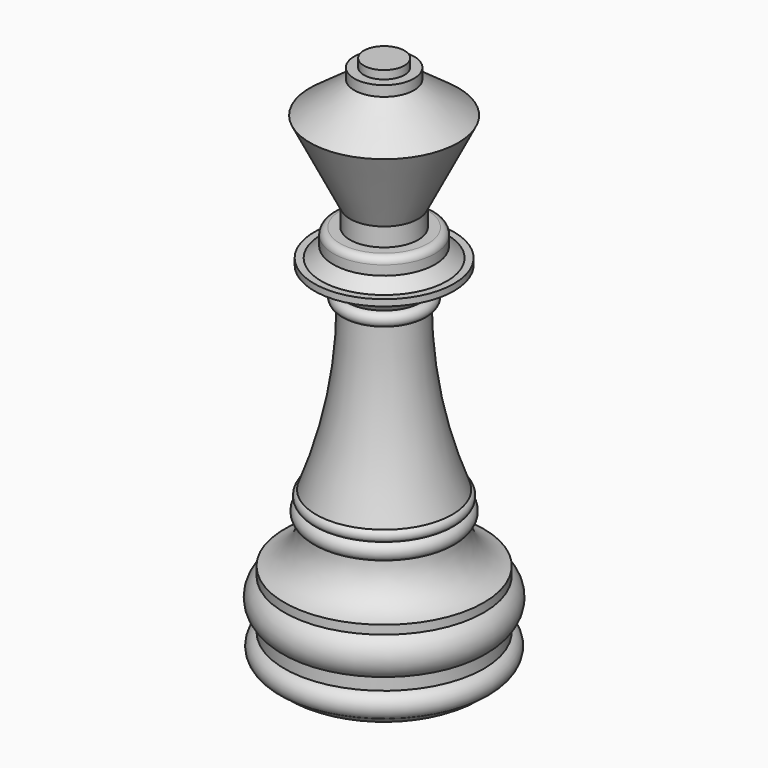
from build123d import *

# Parameters (mm, degrees)
F6_R = 1


# Not quite as in the source:
# - a fillet or chamfer that OpenCascade refuses, or shapes differently, is made with other operations: its cross-section is extruded or revolved along the edge and cut away or added


with BuildPart() as f1:
    # F0 (on Front) → F1 (revolve)
    with BuildSketch(Plane.XZ):
        with BuildLine():
            Line((-200.3652514219, 101.2477203459), (-203.3652514219, 101.2477203459))
            Line((-203.3652514219, 101.2477203459), (-203.3652514219, 21.2477203459))
            Line((-203.3652514219, 21.2477203459), (-188.6436624619, 21.2477203459))
            Line((-188.6436624619, 21.2477203459), (-188.6436624619, 23.0397097766))
            ThreePointArc((-188.6436624619, 23.0397097766), (-187.333962533, 24.8457370326), (-188.6436624619, 26.6517642885))
            Line((-188.6436624619, 26.6517642885), (-188.6436624619, 28.4437537193))
            ThreePointArc((-188.6436624619, 28.4437537193), (-187.1745849151, 31.1942528933), (-188.6436624619, 33.9447520673))
            Line((-188.6436624619, 33.9447520673), (-188.6436624619, 35.2401472628))
            Line((-188.6436624619, 35.2401472628), (-193.309366703, 35.2401472628))
            Line((-193.309366703, 35.2401472628), (-193.309366703, 41.1680191755))
            ThreePointArc((-193.309366703, 41.1680191755), (-192.5565818681, 42.3696450889), (-193.309366703, 43.5712710023))
            ThreePointArc((-193.309366703, 43.5712710023), (-192.8404048548, 44.3696901202), (-193.309366703, 45.1681092381))
            Line((-193.309366703, 45.1681092381), (-197.8608220816, 45.1681092381))
            Line((-197.8608220816, 45.1681092381), (-197.8608220816, 69.3112561437))
            ThreePointArc((-197.8608220816, 69.3112561437), (-196.8800943317, 70.2974423766), (-197.8608220816, 71.2836286096))
            Line((-197.8608220816, 71.2836286096), (-197.8608220816, 74.3284672499))
            Line((-197.8608220816, 74.3284672499), (-193.0439472198, 74.3284672499))
            Line((-193.0439472198, 74.3284672499), (-193.0439472198, 75.2748303938))
            Line((-193.0439472198, 75.2748303938), (-194.0847486258, 75.2748303938))
            Line((-194.0847486258, 75.2748303938), (-195.8655714989, 76.8517457771))
            Line((-195.8655714989, 76.8517457771), (-195.8655714989, 79.2579033303))
            Line((-195.8655714989, 79.2579033303), (-198.3242481947, 79.2579033303))
            Line((-198.3242481947, 79.2579033303), (-198.3242481947, 80.6170105934))
            Line((-198.3242481947, 80.6170105934), (-198.3242481947, 81.9761178565))
            Line((-198.3242481947, 81.9761178565), (-192.4043744802, 93.8070736003))
            Line((-192.4043744802, 93.8070736003), (-198.949098587, 98.5011926961))
            Line((-198.949098587, 98.5011926961), (-198.949098587, 100.0268682092))
            Line((-198.949098587, 100.0268682092), (-200.3652514219, 100.0268682092))
            Line((-200.3652514219, 100.0268682092), (-200.3652514219, 101.2477203459))
        make_face()
    revolve(axis=Axis((-203.3652514219, 0, 61.2477203459), (0, 0, -1)))

    # F2: fillet of radius 5 on 1 edges, made by hand

    # F2_s1 → F2_t2 (revolve, cut)
    with BuildSketch(Plane.XZ):
        with BuildLine():
            ThreePointArc((-188.6436624619, 23.0397097766), (-190.3622558104, 21.7178167682), (-192.4788506174, 21.2477203459))
            Line((-192.4788506174, 21.2477203459), (-188.6436624619, 21.2477203459))
            Line((-188.6436624619, 21.2477203459), (-188.6436624619, 23.0397097766))
        make_face()
    revolve(axis=Axis((-203.3652514219, 0, 21.2477203459), (0, 0, -1)), mode=Mode.SUBTRACT)

    # F3: fillet of radius 6 on 1 edges, made by hand

    # F3_s1 → F3_t2 (revolve)
    with BuildSketch(Plane.XZ):
        with BuildLine():
            ThreePointArc((-193.309366703, 41.0899040806), (-192.0000902375, 37.3486325423), (-188.6436624619, 35.2401472628))
            Line((-188.6436624619, 35.2401472628), (-193.309366703, 35.2401472628))
            Line((-193.309366703, 35.2401472628), (-193.309366703, 41.0899040806))
        make_face()
    revolve(axis=Axis((-203.3652514219, 0, 35.2401472628), (0, 0, -1)))

    # F4: fillet of radius 66.3 on 1 edges, made by hand

    # F4_s1 → F4_t2 (revolve)
    with BuildSketch(Plane.XZ):
        with BuildLine():
            ThreePointArc((-197.8608220816, 69.3095101323), (-196.7130227674, 57.0261577479), (-193.309366703, 45.1681092381))
            Line((-193.309366703, 45.1681092381), (-197.8608220816, 45.1681092381))
            Line((-197.8608220816, 45.1681092381), (-197.8608220816, 69.3095101323))
        make_face()
    revolve(axis=Axis((-203.3652514219, 0, 45.1681092381), (0, 0, -1)))

    # F5: fillet of radius 5.33 on 1 edges, made by hand

    # F5_s1 → F5_t2 (revolve)
    with BuildSketch(Plane.XZ):
        with BuildLine():
            ThreePointArc((-193.0455404117, 74.3284672499), (-195.8941356754, 73.5033984395), (-197.8608220816, 71.2836286096))
            Line((-197.8608220816, 71.2836286096), (-197.8608220816, 74.3284672499))
            Line((-197.8608220816, 74.3284672499), (-193.0455404117, 74.3284672499))
        make_face()
    revolve(axis=Axis((-203.3652514219, 0, 74.3284672499), (0, 0, -1)))

    # F6
    f6_edges = [f1.edges().sort_by_distance(p)[0] for p in [
        (-210.864931, 0, 79.257903),
    ]]
    fillet(f6_edges, radius=F6_R)


solid = f1.part
